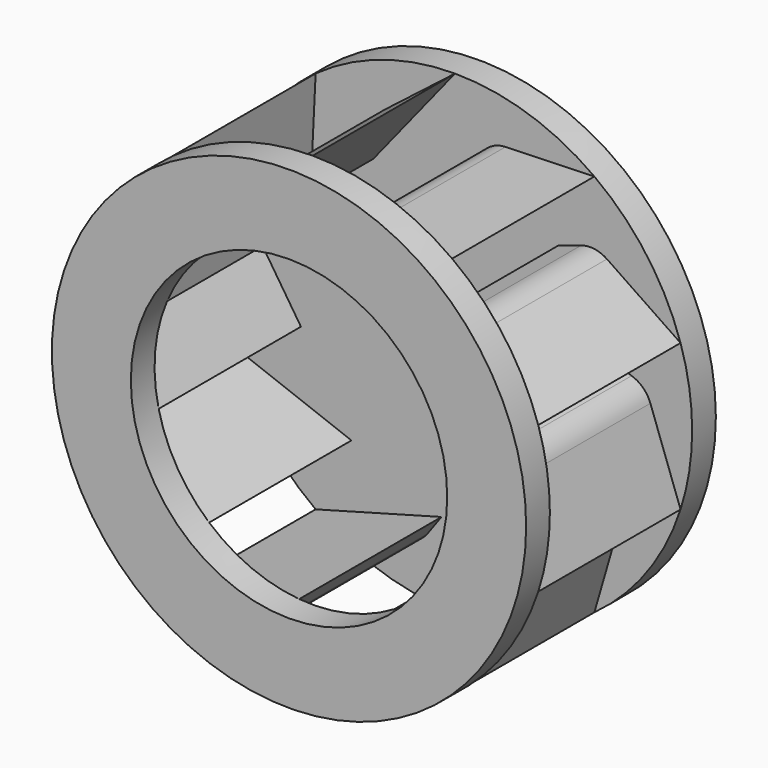
from build123d import *

# Parameters (mm, degrees)
F0_R     = 40
F1_DEPTH = 5
F3_DEPTH = 30
F5_R     = 40
F5_R_2   = 26.6846618965
F6_DEPTH = 5


# Not quite as in the source:
# - the program builds the solid bodies; features that only make, move or delete a surface that nothing else refers to are left out


with BuildPart() as f1:
    # F0 (on Front) → F1 (new body)
    with BuildSketch(Plane.XZ):
        Circle(F0_R)
    extrude(amount=F1_DEPTH)

    # F2 (on face) → F3 (join)
    with BuildSketch(Plane.XZ.offset(5)):
        with BuildLine():
            Line((-13.7807118053, 22.8508897566), (0, 40))
            Line((0, 40), (-11.8473736978, 30.8000143226))
            ThreePointArc((-11.8473736978, 30.8000143226), (-13.2714416715, 29.0493767975), (-13.7807118053, 26.8508897566))
            Line((-13.7807118053, 26.8508897566), (-13.7807118053, 22.8508897566))
        make_face()
        with BuildLine():
            Line((-23.5114100917, 32.360679775), (-27.6885208494, 17.954023476))
            ThreePointArc((-27.6885208494, 17.954023476), (-27.811617122, 15.700681814), (-26.931387055, 13.622726962))
            Line((-26.931387055, 13.622726962), (-24.5802460458, 10.3866589845))
            Line((-24.5802460458, 10.3866589845), (-23.5114100917, 32.360679775))
        make_face()
        with BuildLine():
            Line((-38.0422606518, 12.360679775), (-32.9535941348, -1.7497941036))
            ThreePointArc((-32.9535941348, -1.7497941036), (-31.7287001139, -3.6451399759), (-29.7951878138, -4.8088545127))
            Line((-29.7951878138, -4.8088545127), (-25.9909617486, -6.0449224902))
            Line((-25.9909617486, -6.0449224902), (-38.0422606518, 12.360679775))
        make_face()
        with BuildLine():
            Line((-38.0422606518, -12.360679775), (-25.6315145121, -20.7852498089))
            ThreePointArc((-25.6315145121, -20.7852498089), (-23.5264980812, -21.5986421887), (-21.2782395289, -21.4036170105))
            Line((-21.2782395289, -21.4036170105), (-17.4740134638, -20.167549033))
            Line((-17.4740134638, -20.167549033), (-38.0422606518, -12.360679775))
        make_face()
        with BuildLine():
            Line((-23.5114100917, -32.360679775), (-8.519067529, -31.8814465519))
            ThreePointArc((-8.519067529, -31.8814465519), (-6.3379734177, -31.3021971963), (-4.6337269648, -29.8229252925))
            Line((-4.6337269648, -29.8229252925), (-2.2825859556, -26.586857315))
            Line((-2.2825859556, -26.586857315), (-23.5114100917, -32.360679775))
        make_face()
        with BuildLine():
            Line((0, -40), (11.8473736978, -30.8000143226))
            ThreePointArc((11.8473736978, -30.8000143226), (13.2714416715, -29.0493767975), (13.7807118053, -26.8508897566))
            Line((13.7807118053, -26.8508897566), (13.7807118053, -22.8508897566))
            Line((13.7807118053, -22.8508897566), (0, -40))
        make_face()
        with BuildLine():
            Line((23.5114100917, -32.360679775), (27.6885208494, -17.954023476))
            ThreePointArc((27.6885208494, -17.954023476), (27.811617122, -15.700681814), (26.931387055, -13.622726962))
            Line((26.931387055, -13.622726962), (24.5802460458, -10.3866589845))
            Line((24.5802460458, -10.3866589845), (23.5114100917, -32.360679775))
        make_face()
        with BuildLine():
            Line((38.0422606518, -12.360679775), (32.9535941348, 1.7497941036))
            ThreePointArc((32.9535941348, 1.7497941036), (31.7287001139, 3.6451399759), (29.7951878138, 4.8088545127))
            Line((29.7951878138, 4.8088545127), (25.9909617486, 6.0449224902))
            Line((25.9909617486, 6.0449224902), (38.0422606518, -12.360679775))
        make_face()
        with BuildLine():
            Line((38.0422606518, 12.360679775), (25.6315145121, 20.7852498089))
            ThreePointArc((25.6315145121, 20.7852498089), (23.5264980812, 21.5986421887), (21.2782395289, 21.4036170105))
            Line((21.2782395289, 21.4036170105), (17.4740134638, 20.167549033))
            Line((17.4740134638, 20.167549033), (38.0422606518, 12.360679775))
        make_face()
        with BuildLine():
            Line((23.5114100917, 32.360679775), (8.519067529, 31.8814465519))
            ThreePointArc((8.519067529, 31.8814465519), (6.3379734177, 31.3021971963), (4.6337269648, 29.8229252925))
            Line((4.6337269648, 29.8229252925), (2.2825859556, 26.586857315))
            Line((2.2825859556, 26.586857315), (23.5114100917, 32.360679775))
        make_face()
    extrude(amount=F3_DEPTH)

    # F5 (on offset) → F6 (join)
    with BuildSketch(Plane.XZ.offset(35)):
        Circle(F5_R)
        Circle(F5_R_2, mode=Mode.SUBTRACT)
    extrude(amount=F6_DEPTH)


solid = f1.part
